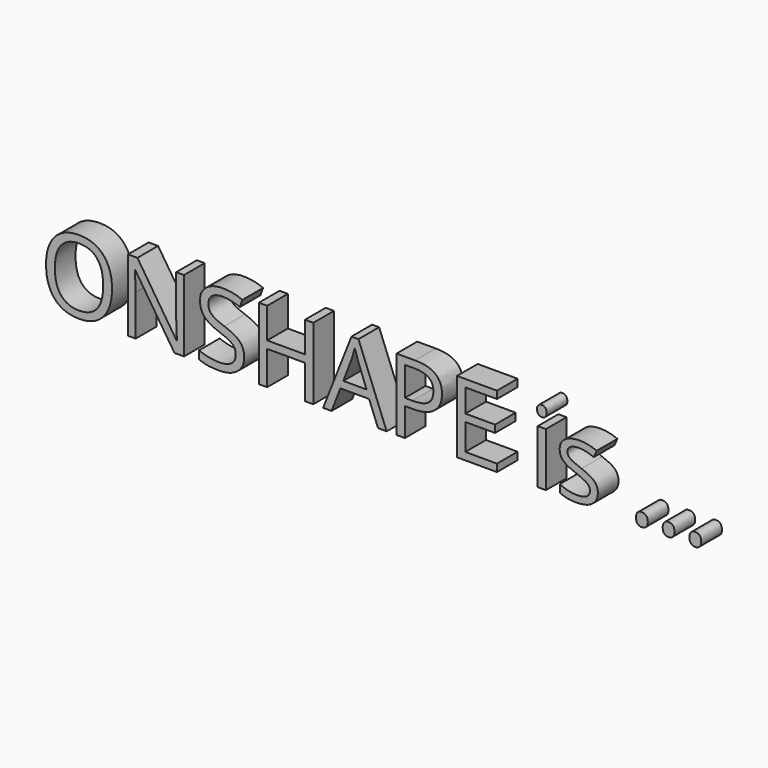
from build123d import *

# Parameters (mm, degrees)
F0_TEXT_SIZE = 98.7188683616
F1_DEPTH     = 25.4


# Not quite as in the source:
# - Text() gives the source's letters only with a copy of the font that has no kerning and outlines rounded to 1/6400 em; it was checked with that copy


with BuildPart() as f1:
    # F0 (on Front) → F1 (new body)
    with BuildSketch(Plane.XZ):
        with Locations((-114.4520565867, -32.7484197915)):
            Text('ONSHAPE is ...', F0_TEXT_SIZE, font='Open Sans', text_align=(TextAlign.LEFT, TextAlign.BOTTOM))
    extrude(amount=F1_DEPTH)


solid = f1.part
